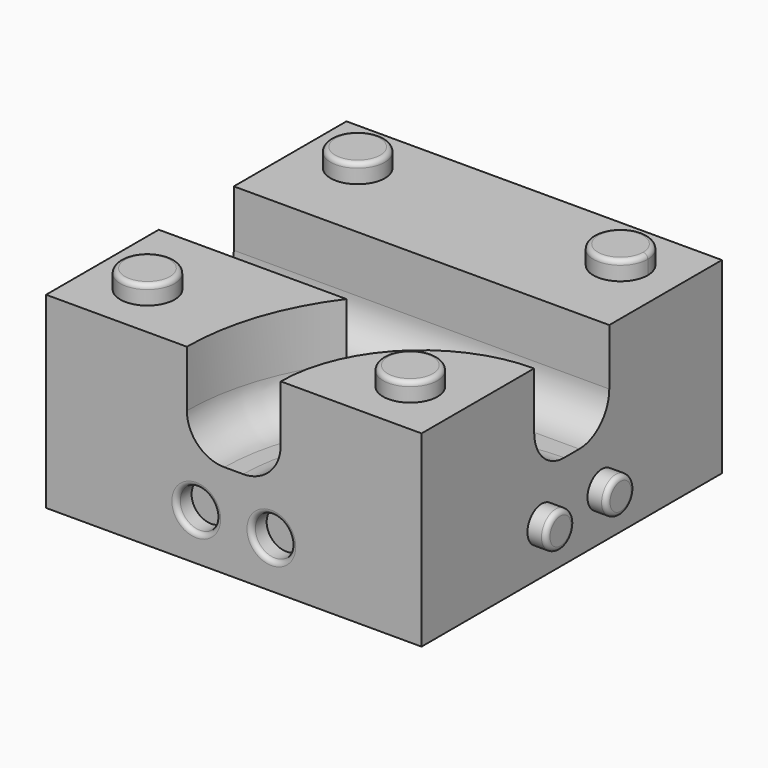
from build123d import *

# Parameters (mm, degrees)
F0_W      = 50.8
F0_H      = 19.05
F0_R      = 3.81
F0_R_2    = 3.683
F1_DEPTH  = 12.7
F0_R_3    = 3.937
F2_DEPTH  = 15.24
F0_R_4    = 5.08
F0_R_5    = 2.667
F0_R_6    = 2.413
F1_FACE_W = 50.8
F1_FACE_H = 19.05
F1_FACE_R = 3.683
F3_DEPTH  = 12.7
F4_START  = -10.16
F4_DEPTH  = 2.54
F7_START  = -22.86
F6_R      = 2.413
F7_DEPTH  = 5.08
F8_START  = 22.86
F6_R_2    = 2.667
F8_DEPTH  = 5.08
F9_START  = 22.86
F5_R      = 2.413
F9_DEPTH  = 5.08
F10_START = -22.86
F5_R_2    = 2.667
F10_DEPTH = 5.08
F11_START = -22.86
F11_DEPTH = 5.08
F12_R     = 5.08
F13_R     = 0.635


with BuildPart() as f1:
    # F0 (on Top) → F1 (new body)
    with BuildSketch(Plane.XY):
        with Locations((0, 15.875)):
            Rectangle(F0_W, F0_H)
        with Locations((-17.78, 17.78)):
            Circle(F0_R, mode=Mode.SUBTRACT)
        with BuildLine():
            ThreePointArc((21.717, 17.78), (14.9961206025, 14.9961206025), (17.78, 21.717))
            ThreePointArc((17.78, 21.717), (20.5638793975, 20.5638793975), (21.717, 17.78))
        make_face(mode=Mode.SUBTRACT)
        with BuildLine():
            ThreePointArc((21.717, 17.78), (20.5638793975, 20.5638793975), (17.78, 21.717))
            ThreePointArc((17.78, 21.717), (14.9961206025, 14.9961206025), (21.717, 17.78))
        make_face()
        with BuildLine():
            ThreePointArc((17.78, 21.463), (20.3842742751, 20.3842742751), (21.463, 17.78))
            ThreePointArc((21.463, 17.78), (15.1757257249, 15.1757257249), (17.78, 21.463))
        make_face(mode=Mode.SUBTRACT)
        with Locations((-17.78, 17.78)):
            Circle(F0_R)
        with Locations((-17.78, 17.78)):
            Circle(F0_R_2, mode=Mode.SUBTRACT)
        with BuildLine():
            ThreePointArc((17.78, 21.463), (15.1757257249, 15.1757257249), (21.463, 17.78))
            ThreePointArc((21.463, 17.78), (20.3842742751, 20.3842742751), (17.78, 21.463))
        make_face()
        with Locations((-17.78, 17.78)):
            Circle(F0_R_2)
    extrude(amount=F1_DEPTH)

    # F0 (on Top) → F2, piece 2 (join)
    with BuildSketch(Plane.XY):
        with Locations((-17.78, 17.78)):
            Circle(F0_R_2)
        with BuildLine():
            ThreePointArc((17.78, 21.463), (15.1757257249, 15.1757257249), (21.463, 17.78))
            ThreePointArc((21.463, 17.78), (20.3842742751, 20.3842742751), (17.78, 21.463))
        make_face()
    extrude(amount=F2_DEPTH)



with BuildPart() as f1b:
    # F0 (on Top) → F1, piece 2 (new body)
    with BuildSketch(Plane.XY):
        with BuildLine():
            Line((25.4, -25.4), (25.4, -6.35))
            ThreePointArc((25.4, -6.35), (11.9296158184, -11.9296158184), (6.35, -25.4))
            Line((6.35, -25.4), (25.4, -25.4))
        make_face()
        with Locations((17.78, -17.78)):
            Circle(F0_R_3, mode=Mode.SUBTRACT)
        with Locations((17.78, -17.78)):
            Circle(F0_R_3)
        with Locations((17.78, -17.78)):
            Circle(F0_R_2, mode=Mode.SUBTRACT)
        with Locations((17.78, -17.78)):
            Circle(F0_R_2)
    extrude(amount=F1_DEPTH)

    # F0 (on Top) → F2, piece 3 (join)
    with BuildSketch(Plane.XY):
        with Locations((17.78, -17.78)):
            Circle(F0_R_2)
    extrude(amount=F2_DEPTH)


with BuildPart() as f1c:
    # F0 (on Top) → F1, piece 3 (new body)
    with BuildSketch(Plane.XY):
        with BuildLine():
            Line((0, -6.35), (-25.4, -6.35))
            Line((-25.4, -6.35), (-25.4, -25.4))
            Line((-25.4, -25.4), (-6.35, -25.4))
            ThreePointArc((-6.35, -25.4), (-4.7206947131, -15.359768429), (0, -6.35))
        make_face()
        with Locations((-17.78, -17.78)):
            Circle(F0_R, mode=Mode.SUBTRACT)
        with Locations((-17.78, -17.78)):
            Circle(F0_R)
        with Locations((-17.78, -17.78)):
            Circle(F0_R_2, mode=Mode.SUBTRACT)
        with Locations((-17.78, -17.78)):
            Circle(F0_R_2)
    extrude(amount=F1_DEPTH)

    # F0 (on Top) → F2 (join)
    with BuildSketch(Plane.XY):
        with Locations((-17.78, -17.78)):
            Circle(F0_R_2)
    extrude(amount=F2_DEPTH)


with BuildPart() as f1_1:
    add(f1.part)

    add(f1b.part)  # F3 merges F1b

    add(f1c.part)  # F3 merges F1c
    # F0 (on Top) + F1_face (on face) → F3 (join)
    with BuildSketch(Plane.XY):
        with Locations((0, 15.875)):
            Rectangle(F0_W, F0_H)
        with Locations((-17.78, 17.78)):
            Circle(F0_R, mode=Mode.SUBTRACT)
        with BuildLine():
            ThreePointArc((21.717, 17.78), (14.9961206025, 14.9961206025), (17.78, 21.717))
            ThreePointArc((17.78, 21.717), (20.5638793975, 20.5638793975), (21.717, 17.78))
        make_face(mode=Mode.SUBTRACT)
        with BuildLine():
            Line((25.4, -6.35), (25.4, 6.35))
            Line((25.4, 6.35), (-25.4, 6.35))
            Line((-25.4, 6.35), (-25.4, -6.35))
            Line((-25.4, -6.35), (0, -6.35))
            ThreePointArc((0, -6.35), (-4.7206947131, -15.359768429), (-6.35, -25.4))
            Line((-6.35, -25.4), (6.35, -25.4))
            ThreePointArc((6.35, -25.4), (11.9296158184, -11.9296158184), (25.4, -6.35))
        make_face()
        Circle(F0_R_4, mode=Mode.SUBTRACT)
        with BuildLine():
            Line((0, -6.35), (-25.4, -6.35))
            Line((-25.4, -6.35), (-25.4, -25.4))
            Line((-25.4, -25.4), (-6.35, -25.4))
            ThreePointArc((-6.35, -25.4), (-4.7206947131, -15.359768429), (0, -6.35))
        make_face()
        with Locations((-17.78, -17.78)):
            Circle(F0_R, mode=Mode.SUBTRACT)
        with BuildLine():
            Line((25.4, -25.4), (25.4, -6.35))
            ThreePointArc((25.4, -6.35), (11.9296158184, -11.9296158184), (6.35, -25.4))
            Line((6.35, -25.4), (25.4, -25.4))
        make_face()
        with Locations((17.78, -17.78)):
            Circle(F0_R_3, mode=Mode.SUBTRACT)
        Circle(F0_R_4)
        Circle(F0_R_5, mode=Mode.SUBTRACT)
        with BuildLine():
            ThreePointArc((21.717, 17.78), (20.5638793975, 20.5638793975), (17.78, 21.717))
            ThreePointArc((17.78, 21.717), (14.9961206025, 14.9961206025), (21.717, 17.78))
        make_face()
        with BuildLine():
            ThreePointArc((17.78, 21.463), (20.3842742751, 20.3842742751), (21.463, 17.78))
            ThreePointArc((21.463, 17.78), (15.1757257249, 15.1757257249), (17.78, 21.463))
        make_face(mode=Mode.SUBTRACT)
        with Locations((17.78, -17.78)):
            Circle(F0_R_3)
        with Locations((17.78, -17.78)):
            Circle(F0_R_2, mode=Mode.SUBTRACT)
        with Locations((-17.78, -17.78)):
            Circle(F0_R)
        with Locations((-17.78, -17.78)):
            Circle(F0_R_2, mode=Mode.SUBTRACT)
        with Locations((-17.78, 17.78)):
            Circle(F0_R)
        with Locations((-17.78, 17.78)):
            Circle(F0_R_2, mode=Mode.SUBTRACT)
        with Locations((-17.78, -17.78)):
            Circle(F0_R_2)
        with Locations((-17.78, 17.78)):
            Circle(F0_R_2)
        with BuildLine():
            ThreePointArc((17.78, 21.463), (15.1757257249, 15.1757257249), (21.463, 17.78))
            ThreePointArc((21.463, 17.78), (20.3842742751, 20.3842742751), (17.78, 21.463))
        make_face()
        with Locations((17.78, -17.78)):
            Circle(F0_R_2)
        Circle(F0_R_5)
        Circle(F0_R_6, mode=Mode.SUBTRACT)
        Circle(F0_R_6)
    with BuildSketch(Plane(origin=(0, 15.6910254438, 12.7), x_dir=(1, 0, 0), z_dir=(0, 0, 1))):
        with Locations((0, 0.1839745562)):
            Rectangle(F1_FACE_W, F1_FACE_H)
        with Locations((-17.78, 2.0889745562)):
            Circle(F1_FACE_R, mode=Mode.SUBTRACT)
        with Locations((17.78, 2.0889745562)):
            Circle(F1_FACE_R, mode=Mode.SUBTRACT)
    extrude(amount=-F3_DEPTH)

    # F0 (on Top) → F4 (cut)
    with BuildSketch(Plane.XY.offset(F4_START)):
        with Locations((17.78, -17.78)):
            Circle(F0_R_3)
        with Locations((17.78, -17.78)):
            Circle(F0_R_2, mode=Mode.SUBTRACT)
        with BuildLine():
            ThreePointArc((21.717, 17.78), (20.5638793975, 20.5638793975), (17.78, 21.717))
            ThreePointArc((17.78, 21.717), (14.9961206025, 14.9961206025), (21.717, 17.78))
        make_face()
        with BuildLine():
            ThreePointArc((17.78, 21.463), (20.3842742751, 20.3842742751), (21.463, 17.78))
            ThreePointArc((21.463, 17.78), (15.1757257249, 15.1757257249), (17.78, 21.463))
        make_face(mode=Mode.SUBTRACT)
        with Locations((-17.78, -17.78)):
            Circle(F0_R)
        with Locations((-17.78, -17.78)):
            Circle(F0_R_2, mode=Mode.SUBTRACT)
        with Locations((-17.78, 17.78)):
            Circle(F0_R)
        with Locations((-17.78, 17.78)):
            Circle(F0_R_2, mode=Mode.SUBTRACT)
        with Locations((-17.78, -17.78)):
            Circle(F0_R_2)
        with Locations((-17.78, 17.78)):
            Circle(F0_R_2)
        with BuildLine():
            ThreePointArc((17.78, 21.463), (15.1757257249, 15.1757257249), (21.463, 17.78))
            ThreePointArc((21.463, 17.78), (20.3842742751, 20.3842742751), (17.78, 21.463))
        make_face()
        with Locations((17.78, -17.78)):
            Circle(F0_R_2)
    extrude(amount=-F4_DEPTH, mode=Mode.SUBTRACT)

    # F6 (on Front) → F7 (join)
    with BuildSketch(Plane.XZ.offset(F7_START)):
        with Locations((-5.08, -6.35)):
            Circle(F6_R)
    extrude(amount=-F7_DEPTH)

    # F6 (on Front) → F8 (cut)
    with BuildSketch(Plane.XZ.offset(F8_START)):
        with Locations((-5.08, -6.35)):
            Circle(F6_R_2)
        with Locations((-5.08, -6.35)):
            Circle(F6_R, mode=Mode.SUBTRACT)
        with Locations((5.08, -6.35)):
            Circle(F6_R_2)
        with Locations((5.08, -6.35)):
            Circle(F6_R, mode=Mode.SUBTRACT)
        with Locations((-5.08, -6.35)):
            Circle(F6_R)
        with Locations((5.08, -6.35)):
            Circle(F6_R)
    extrude(amount=F8_DEPTH, mode=Mode.SUBTRACT)

    # F5 (on Right) → F9 (join)
    with BuildSketch(Plane.YZ.offset(F9_START)):
        with Locations((-5.08, -6.35)):
            Circle(F5_R)
        with Locations((5.08, -6.35)):
            Circle(F5_R)
    extrude(amount=F9_DEPTH)

    # F5 (on Right) → F10 (cut)
    with BuildSketch(Plane.YZ.offset(F10_START)):
        with Locations((-5.08, -6.35)):
            Circle(F5_R_2)
        with Locations((-5.08, -6.35)):
            Circle(F5_R, mode=Mode.SUBTRACT)
        with Locations((5.08, -6.35)):
            Circle(F5_R_2)
        with Locations((5.08, -6.35)):
            Circle(F5_R, mode=Mode.SUBTRACT)
        with Locations((-5.08, -6.35)):
            Circle(F5_R)
        with Locations((5.08, -6.35)):
            Circle(F5_R)
    extrude(amount=-F10_DEPTH, mode=Mode.SUBTRACT)

    # F6 (on Front) → F11 (cut)
    with BuildSketch(Plane.XZ.offset(F11_START)):
        with Locations((5.08, -6.35)):
            Circle(F6_R_2)
        with Locations((5.08, -6.35)):
            Circle(F6_R, mode=Mode.SUBTRACT)
        with Locations((5.08, -6.35)):
            Circle(F6_R)
    extrude(amount=-F11_DEPTH, mode=Mode.SUBTRACT)

    # F12
    f12_edges = [f1_1.edges().sort_by_distance(p)[0] for p in [
        (11.929616, -11.929616, 0),
        (0, 6.35, 0),
        (-4.720695, -15.359768, 0),
        (-12.7, -6.35, 0),
    ]]
    fillet(f12_edges, radius=F12_R)

    # F13
    f13_edges = [f1_1.edges().sort_by_distance(p)[0] for p in [
        (-21.463, -17.78, 15.24),
        (-21.463, 17.78, 15.24),
        (-7.493, 27.94, -6.35),
        (-25.4, -7.747, -6.35),
        (27.94, 2.667, -6.35),
        (27.94, -7.493, -6.35),
        (-25.4, 2.413, -6.35),
        (14.097, 17.78, 15.24),
        (14.097, -17.78, 15.24),
        (13.843, -17.78, -12.7),
        (17.78, 13.843, -12.7),
        (-21.59, 17.78, -12.7),
        (-21.59, -17.78, -12.7),
        (-7.747, -25.4, -6.35),
        (2.413, -25.4, -6.35),
        (2.413, 25.4, -6.35),
    ]]
    fillet(f13_edges, radius=F13_R)


solid = f1_1.part
